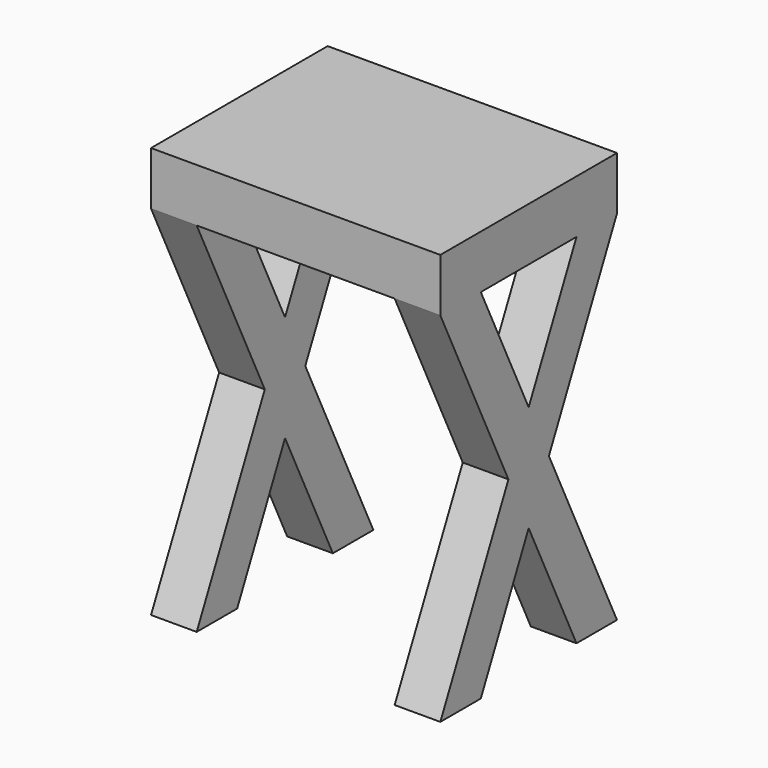
from build123d import *

# Parameters (mm, degrees)
F0_W     = 482.6
F0_H     = 368.3
F1_DEPTH = 88.9
F3_DEPTH = 482.6
F4_W     = 330.2
F4_H     = 596.9
F5_DEPTH = 368.301


with BuildPart() as f1:
    # F0 (on Top) → F1 (new body)
    with BuildSketch(Plane.XY):
        Rectangle(F0_W, F0_H)
    extrude(amount=F1_DEPTH)

    # F2 (on face) → F3 (join)
    with BuildSketch(Plane.YZ.offset(241.3)):
        Polygon((-99.7690824552, 0), (-184.15, 0), (-42.1904587724, -298.45), (0, -209.7504852528), align=None)
        Polygon((99.7690824552, 0), (0, -209.7504852528), (42.1904587724, -298.45), (184.15, 0), align=None)
        Polygon((0, -209.7504852528), (-42.1904587724, -298.45), (0, -387.1495147472), (42.1904587724, -298.45), align=None)
        Polygon((42.1904587724, -298.45), (0, -387.1495147472), (99.7690824552, -596.9), (184.15, -596.9), align=None)
        Polygon((0, -387.1495147472), (-42.1904587724, -298.45), (-184.15, -596.9), (-99.7690824552, -596.9), align=None)
    extrude(amount=-F3_DEPTH)

    # F4 (on face) → F5 (cut, through all)
    with BuildSketch(Plane(origin=(0, 184.15, 0), x_dir=(-1, 0, 0), z_dir=(0, 1, 0))):
        with Locations((0, -298.45)):
            Rectangle(F4_W, F4_H)
    extrude(amount=-F5_DEPTH, mode=Mode.SUBTRACT)


solid = f1.part
